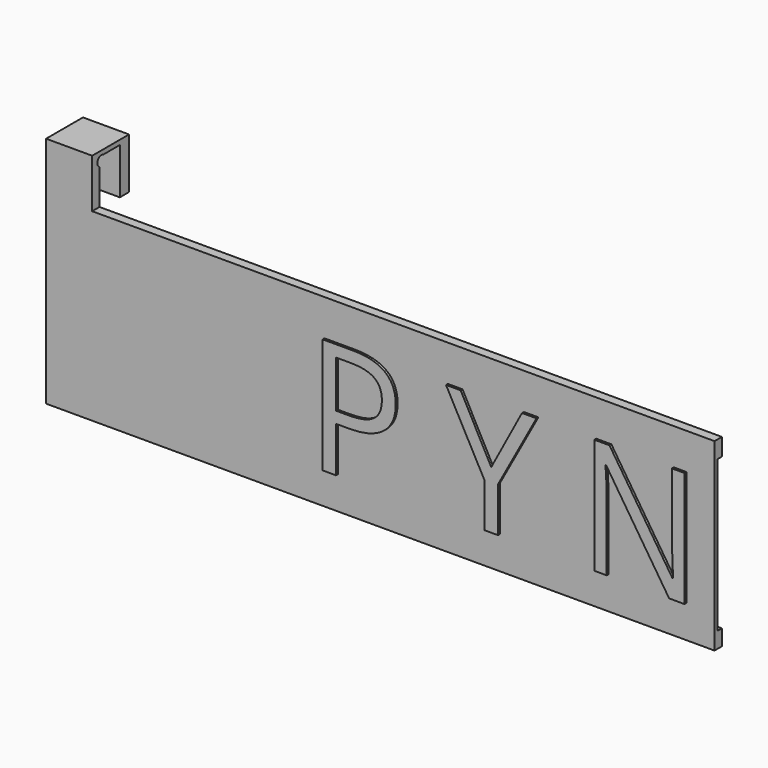
from build123d import *

# Parameters (mm, degrees)
F1_TEXT_SIZE = 44.5169422569
F2_DEPTH     = 0.635
F0_W         = 184.15
F0_H         = 50.8
F3_DEPTH     = 2.54
F4_W         = 184.15
F4_H         = 13.0136748776
F5_DEPTH     = 1.4478
F6_W         = 12.7
F6_H         = 2.54
F7_DEPTH     = 13.462
F8_W         = 12.7
F8_H         = 1.2703451927
F9_DEPTH     = 10.16
F10_W        = 12.7
F10_H        = 3.1772071168
F11_DEPTH    = 12.7
F12_W        = 19.0491899848
F12_H        = 41.6447743773
F13_DEPTH    = 13.208
F14_R        = 1.3841754701
F15_DEPTH    = 25.4


# Not quite as in the source:
# - Text() gives the source's letters only with a copy of the font that has no kerning and outlines rounded to 1/6400 em; it was checked with that copy


with BuildPart() as f2:
    # F1 (on face) → F2 (new body, symmetric)
    with BuildSketch(Plane.XZ):
        with Locations((-19.7615064681, -16.3875905564)):
            Text('P Y N', F1_TEXT_SIZE, font='Open Sans', text_align=(TextAlign.LEFT, TextAlign.BOTTOM))
    extrude(amount=F2_DEPTH, both=True)


with BuildPart() as f3:
    # F0 (on Front) → F3 (new body)
    with BuildSketch(Plane.XZ):
        Rectangle(F0_W, F0_H)
    extrude(amount=-F3_DEPTH)

    # F4 (on face) → F5 (cut)
    with BuildSketch(Plane(origin=(0, 2.54, 0), x_dir=(-1, 0, 0), z_dir=(0, 1, 0))):
        Rectangle(F4_W, F4_H)
    extrude(amount=-F5_DEPTH, mode=Mode.SUBTRACT)

    # F6 (on face) → F7 (join)
    with BuildSketch(Plane.XY.offset(25.4)):
        with Locations((-85.725, 1.27)):
            Rectangle(F6_W, F6_H)
    extrude(amount=F7_DEPTH)

    # F8 (on face) → F9 (join)
    with BuildSketch(Plane(origin=(0, 2.54, 0), x_dir=(-1, 0, 0), z_dir=(0, 1, 0))):
        with Locations((85.725, 38.2268274037)):
            Rectangle(F8_W, F8_H)
    extrude(amount=F9_DEPTH)

    # F10 (on face) → F11 (join)
    with BuildSketch(Plane(origin=(0, 0, 37.5916548073), x_dir=(1, 0, 0), z_dir=(0, 0, -1))):
        with Locations((-85.725, -11.1113964416)):
            Rectangle(F10_W, F10_H)
    extrude(amount=F11_DEPTH)

    # F12 (on face) → F13 (cut)
    with BuildSketch(Plane(origin=(0, 1.0922, 0), x_dir=(-1, 0, 0), z_dir=(0, 1, 0))):
        with Locations((-82.6691053808, -0.2066679299)):
            Rectangle(F12_W, F12_H)
    extrude(amount=F13_DEPTH, mode=Mode.SUBTRACT)

    # F14 (on face) → F15 (cut)
    with BuildSketch(Plane(origin=(-92.075, 0, 0), x_dir=(0, -1, 0), z_dir=(-1, 0, 0))):
        with Locations((-3.1707454473, 36.3512039185)):
            Circle(F14_R)
    extrude(amount=-F15_DEPTH, mode=Mode.SUBTRACT)


solid = Compound([f2.part, f3.part])
